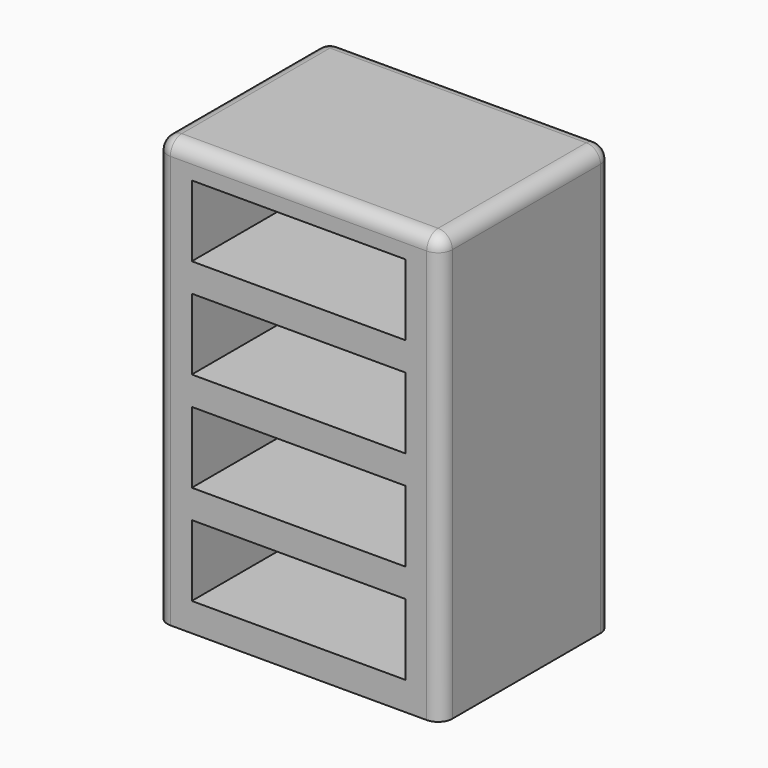
from build123d import *

# Parameters (mm, degrees)
F0_W         = 101.6
F0_H         = 76.2
F1_DEPTH     = 152.4
F2_W         = 76.2
F2_H         = 25.4
F3_DEPTH     = 64.77
F4_R         = 5.08
F5_R         = 5.08
F6_T1_DEPTH  = 160.02
F6_S5_W      = 5.08
F6_S5_H      = 5.08
F6_T6_DEPTH  = 5.08
F6_S11_W     = 5.08
F6_S11_H     = 5.08
F6_T12_DEPTH = 5.08


# Not quite as in the source:
# - a fillet or chamfer that OpenCascade refuses, or shapes differently, is made with other operations: its cross-section is extruded or revolved along the edge and cut away or added


with BuildPart() as f1:
    # F0 (on Top) → F1 (new body)
    with BuildSketch(Plane.XY):
        with Locations((-50.8, 38.1)):
            Rectangle(F0_W, F0_H)
    extrude(amount=F1_DEPTH)

    # F2 (on face) → F3 (cut)
    with BuildSketch(Plane.XZ):
        with Locations((-50.8, 129.54)):
            Rectangle(F2_W, F2_H)
        with Locations((-50.8, 93.98)):
            Rectangle(F2_W, F2_H)
        with Locations((-50.8, 58.42)):
            Rectangle(F2_W, F2_H)
        with Locations((-50.8, 22.86)):
            Rectangle(F2_W, F2_H)
    extrude(amount=-F3_DEPTH, mode=Mode.SUBTRACT)

    # F4
    f4_edges = [f1.edges().sort_by_distance(p)[0] for p in [
        (-50.8, 0, 152.4),
        (-101.6, 38.1, 152.4),
    ]]
    fillet(f4_edges, radius=F4_R)

    # F5
    f5_edges = [f1.edges().sort_by_distance(p)[0] for p in [
        (0, 40.64, 152.4),
        (-48.26, 76.2, 152.4),
    ]]
    fillet(f5_edges, radius=F5_R)

    # F6: fillet of radius 5.08 on 2 edges, made by hand

    # F6_s2 → F6_t1 (cut)
    with BuildSketch(Plane.XY.offset(-12.7)):
        with BuildLine():
            ThreePointArc((0, 71.12), (-1.4878975516, 74.7121024484), (-5.08, 76.2))
            Line((-5.08, 76.2), (0, 76.2))
            Line((0, 76.2), (0, 71.12))
        make_face()
        with BuildLine():
            ThreePointArc((-96.52, 0), (-100.1121024484, 1.4878975516), (-101.6, 5.08))
            Line((-101.6, 5.08), (-101.6, 0))
            Line((-101.6, 0), (-96.52, 0))
        make_face()
    extrude(amount=F6_T1_DEPTH, mode=Mode.SUBTRACT)


with BuildPart() as f6_tool4:
    # F6_s5 → F6_t6 (new body)
    with BuildSketch(Plane.XZ.offset(-5.08)):
        with Locations((-99.06, 149.86)):
            Rectangle(F6_S5_W, F6_S5_H)
    extrude(amount=F6_T6_DEPTH)

    # F6_s7 → F6_t8 (revolve, cut)
    with BuildSketch(Plane(origin=(-96.52, 5.08, 147.32), x_dir=(0.7071067812, 0, -0.7071067812), z_dir=(-0.7071067812, 0, -0.7071067812))):
        with BuildLine():
            ThreePointArc((0, -5.08), (5.08, 0), (0, 5.08))
            Line((0, 5.08), (0, -5.08))
        make_face()
    revolve(axis=Axis((-96.52, 5.08, 147.32), (0, -1, 0)), mode=Mode.SUBTRACT)


with BuildPart() as f1_1:
    add(f1.part)

    # F6_t3: cut F6_tool4
    add(f6_tool4.part, mode=Mode.SUBTRACT)


with BuildPart() as f6_tool10:
    # F6_s11 → F6_t12 (new body)
    with BuildSketch(Plane.YZ.offset(-5.08)):
        with Locations((73.66, 149.86)):
            Rectangle(F6_S11_W, F6_S11_H)
    extrude(amount=F6_T12_DEPTH)

    # F6_s13 → F6_t14 (revolve, cut)
    with BuildSketch(Plane(origin=(-5.08, 71.12, 147.32), x_dir=(0, -0.7071067812, -0.7071067812), z_dir=(0, -0.7071067812, 0.7071067812))):
        with BuildLine():
            ThreePointArc((0, -5.08), (5.08, 0), (0, 5.08))
            Line((0, 5.08), (0, -5.08))
        make_face()
    revolve(axis=Axis((-5.08, 71.12, 147.32), (1, 0, 0)), mode=Mode.SUBTRACT)


with BuildPart() as f1_2:
    add(f1_1.part)

    # F6_t9: cut F6_tool10
    add(f6_tool10.part, mode=Mode.SUBTRACT)


solid = f1_2.part
